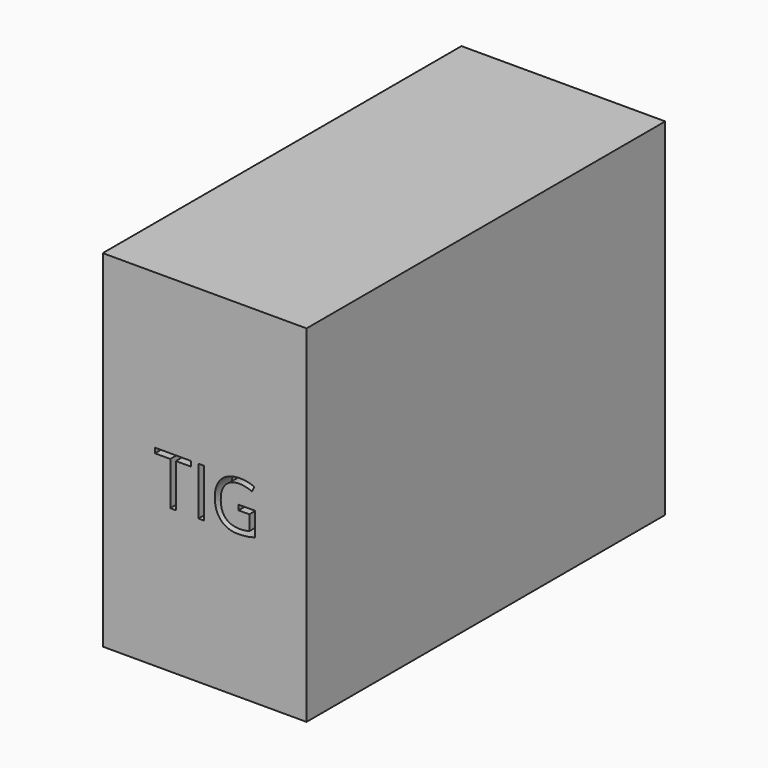
from build123d import *

# Parameters (mm, degrees)
F0_W         = 254
F0_H         = 431.8
F1_DEPTH     = 558.8
F2_TEXT_SIZE = 84.3270203414
F3_DEPTH     = 25.4


# Not quite as in the source:
# - Text() gives the source's letters only with a copy of the font that has no kerning and outlines rounded to 1/6400 em; it was checked with that copy


with BuildPart() as f1:
    # F0 (on Front) → F1 (new body)
    with BuildSketch(Plane.XZ):
        Rectangle(F0_W, F0_H)
    extrude(amount=-F1_DEPTH)

    # F2 (on face) → F3 (cut)
    with BuildSketch(Plane.XZ):
        with Locations((-62.6918691851, -36.5901999176)):
            Text('TIG', F2_TEXT_SIZE, font='Open Sans', text_align=(TextAlign.LEFT, TextAlign.BOTTOM))
    extrude(amount=-F3_DEPTH, mode=Mode.SUBTRACT)


solid = f1.part
